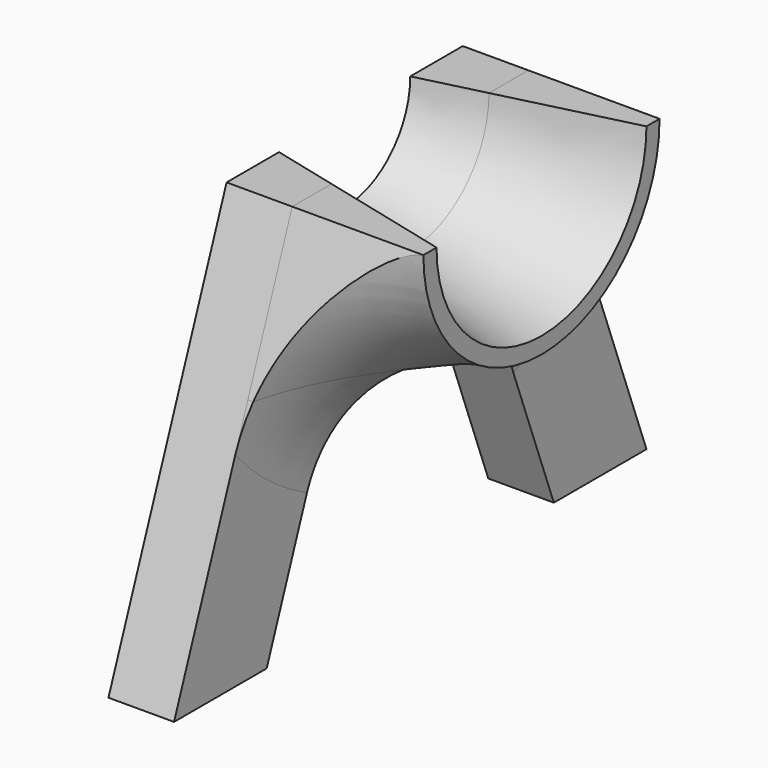
from build123d import *

# Parameters (mm, degrees)
F1_DEPTH     = 12.7
F6_ANGLE     = 180
F7_T4_ANGLE  = 90.0000003922
F7_T10_ANGLE = 227.9415431295
F7_T17_ANGLE = 89.9999996078
F7_T23_ANGLE = 89.9999996078


# Not quite as in the source:
# - a fillet or chamfer that OpenCascade refuses, or shapes differently, is made with other operations: its cross-section is extruded or revolved along the edge and cut away or added


with BuildPart() as f1:
    # F0 (on Right) → F1 (new body)
    with BuildSketch(Plane.YZ):
        with BuildLine():
            Line((-57.16524, 0), (-34.7472, 0))
            Line((-34.7472, 0), (-16.8783, 47.625))
            Line((-16.8783, 47.625), (0, 47.625))
            Line((0, 47.625), (0, 60.325))
            ThreePointArc((0, 60.325), (-11.2253201513, 64.9746798487), (-15.875, 76.2))
            Line((-15.875, 76.2), (-28.575, 76.2))
            Line((-28.575, 76.2), (-57.16524, 0))
        make_face()
    extrude(amount=F1_DEPTH)

    # F2: F1 across plane


with BuildPart() as f1_1:
    add(f1.part)
    add(f1.part.mirror(Plane.XZ))

    # F3 (on face) → F4 (revolve, cut)
    with BuildSketch(Plane.XY.offset(76.2)):
        Polygon((12.7, -15.875), (0, -15.875), (12.7, -19.05), align=None)
    revolve(axis=Axis((5.5597093888, 0, 76.2), (-1, 0, 0)), mode=Mode.SUBTRACT)

    # F5 (on face) → F6 (revolve)
    with BuildSketch(Plane.XY.offset(76.2)):
        Polygon((38.1, -25.4), (12.7, -19.05), (12.7, -28.575), (38.1, -28.575), align=None)
    revolve(axis=Axis((19.4450803101, 0, 76.2), (1, 0, 0)), revolution_arc=F6_ANGLE)

    # F7: fillet of radius 27.5944610179 on 1 edges, made by hand


with BuildPart() as f7_tool2:
    # F7_s3 → F7_t4 (revolve)
    with BuildSketch(Plane.XY.offset(76.2)):
        with BuildLine():
            ThreePointArc((12.7, -56.0820649054), (20.0212120444, -37.3617642954), (38.1, -28.575))
            Line((38.1, -28.575), (12.7, -28.575))
            Line((12.7, -28.575), (12.7, -56.0820649054))
        make_face()
    revolve(axis=Axis((12.7, 0, 76.2), (1, 0, 0)), revolution_arc=F7_T4_ANGLE)

    split(bisect_by=Plane(origin=(0, -50.1108790038, 18.8016018022), x_dir=(1, 0, 0), z_dir=(0, 0.9362676004, -0.3512876037)), keep=Keep.TOP)

    split(bisect_by=Plane.XY.offset(47.625), keep=Keep.TOP)


with BuildPart() as f1_2:
    add(f1_1.part)

    # F7_t1: union F7_tool2
    add(f7_tool2.part)


with BuildPart() as f7_tool8:
    # F7_s9 → F7_t10 (revolve)
    with BuildSketch(Plane(origin=(0, -37.8993318562, 42.0052074025), x_dir=(1, 0, 0), z_dir=(0, 0.6698884676, -0.7424617438))):
        with BuildLine():
            ThreePointArc((12.7, -107.1275661365), (20.0212120444, -88.4072655265), (38.1, -79.6205012311))
            Line((38.1, -79.6205012311), (12.7, -79.6205012311))
            Line((12.7, -79.6205012311), (12.7, -107.1275661365))
        make_face()
    revolve(axis=Axis((12.7, 0, 76.2), (1, 0, 0)), revolution_arc=F7_T10_ANGLE)

    split(bisect_by=Plane(origin=(0, -50.1108790038, 18.8016018022), x_dir=(1, 0, 0), z_dir=(0, 0.9362676004, -0.3512876037)), keep=Keep.TOP)

    split(bisect_by=Plane(origin=(0, -30.4592919565, 11.4283263421), x_dir=(1, 0, 0), z_dir=(0, -0.9362676004, 0.3512876037)), keep=Keep.TOP)

    split(bisect_by=Plane.XY.offset(47.625), keep=Keep.BOTTOM)


with BuildPart() as f1_3:
    add(f1_2.part)

    # F7_t7: union F7_tool8
    add(f7_tool8.part)


with BuildPart() as f7_tool15:
    # F7_s16 → F7_t17 (revolve)
    with BuildSketch(Plane.XZ):
        with BuildLine():
            ThreePointArc((38.1, 47.625), (20.0212120444, 38.8382357046), (12.7, 20.1179350946))
            Line((12.7, 20.1179350946), (12.7, 47.625))
            Line((12.7, 47.625), (38.1, 47.625))
        make_face()
    revolve(axis=Axis((12.7, 0, 76.2), (1, 0, 0)), revolution_arc=F7_T17_ANGLE)

    split(bisect_by=Plane.XY.offset(47.625), keep=Keep.TOP)

    split(bisect_by=Plane(origin=(0, 50.1108790038, 18.8016018022), x_dir=(1, 0, 0), z_dir=(0, -0.9362676004, -0.3512876037)), keep=Keep.TOP)


with BuildPart() as f1_4:
    add(f1_3.part)

    # F7_t14: union F7_tool15
    add(f7_tool15.part)


with BuildPart() as f7_tool21:
    # F7_s22 → F7_t23 (revolve)
    with BuildSketch(Plane.XZ):
        with BuildLine():
            ThreePointArc((38.1, 47.625), (20.0212120444, 38.8382357046), (12.7, 20.1179350946))
            Line((12.7, 20.1179350946), (12.7, 47.625))
            Line((12.7, 47.625), (38.1, 47.625))
        make_face()
    revolve(axis=Axis((12.7, 0, 76.2), (1, 0, 0)), revolution_arc=F7_T23_ANGLE)

    split(bisect_by=Plane(origin=(0, 30.4592919565, 11.4283263421), x_dir=(1, 0, 0), z_dir=(0, 0.9362676004, 0.3512876037)), keep=Keep.TOP)

    split(bisect_by=Plane(origin=(0, 50.1108790038, 18.8016018022), x_dir=(1, 0, 0), z_dir=(0, -0.9362676004, -0.3512876037)), keep=Keep.TOP)


with BuildPart() as f1_5:
    add(f1_4.part)

    # F7_t20: union F7_tool21
    add(f7_tool21.part)


solid = f1_5.part
